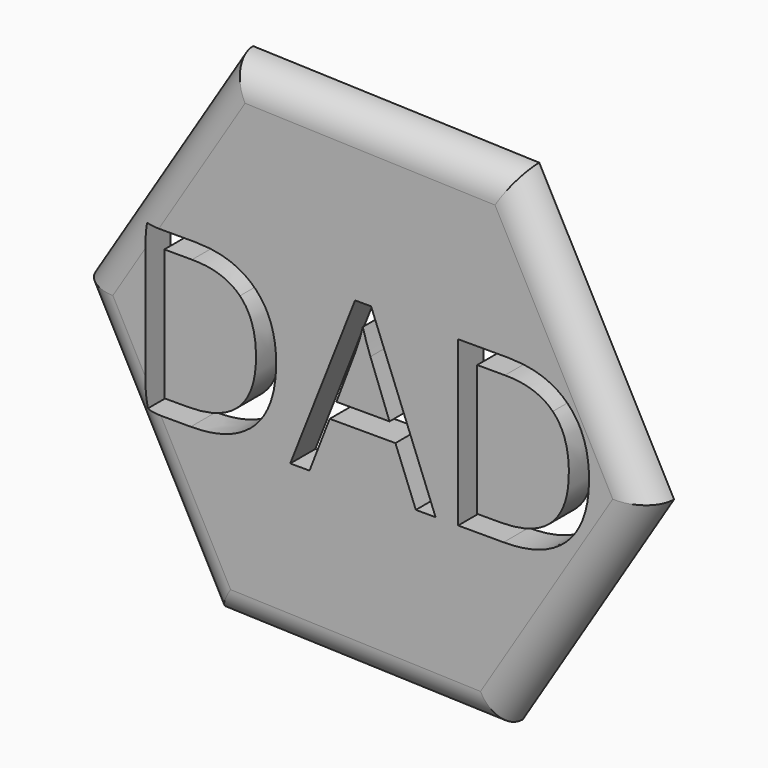
from build123d import *

# Parameters (mm, degrees)
F1_DEPTH     = 5
F2_T1_DEPTH  = 70.5879001638
F2_T3_DEPTH  = 70.5879001638
F2_T5_DEPTH  = 70.5879001638
F2_T7_DEPTH  = 70.5879001638
F2_T9_DEPTH  = 70.5879001638
F2_T11_DEPTH = 70.5879001638


# Not quite as in the source:
# - a fillet or chamfer that OpenCascade refuses, or shapes differently, is made with other operations: its cross-section is extruded or revolved along the edge and cut away or added


with BuildPart() as f1:
    # F0 (on Front) → F1 (new body)
    with BuildSketch(Plane.XZ):
        with BuildLine():
            Line((-4.1963754653, -1.9962660098), (4.2509359723, -1.9962660098))
            Line((4.2509359723, -1.9962660098), (1.2103610841, 6.0966927153))
            add(Edge.make_bspline(
                [(1.2103610841, 6.0966927153), (0.621678352, 7.6341262584), (-0.0012965781, 9.8631191276)],
                knots=[0, 0, 0, 1, 1, 1], degree=2))
            add(Edge.make_bspline(
                [(-0.0012965781, 9.8631191276), (-0.395656855, 8.1485092282), (-1.1272237454, 6.0966927153)],
                knots=[0, 0, 0, 1, 1, 1], degree=2))
            Line((-1.1272237454, 6.0966927153), (-4.1963754653, -1.9962660098))
        make_face()
    extrude(amount=F1_DEPTH)


with BuildPart() as f1b:
    # F0 (on Front) → F1, piece 2 (new body)
    with BuildSketch(Plane.XZ):
        with BuildLine():
            add(Edge.make_bspline(
                [(30.0758187402, -7.7373514895), (32.8106215297, -5.0654177297), (32.8106215297, 0.1641424634)],
                knots=[0, 0, 0, 1, 1, 1], degree=2))
            add(Edge.make_bspline(
                [(32.8106215297, 0.1641424634), (32.8106215297, 5.2736799636), (30.2472797301, 7.8627409117)],
                knots=[0, 0, 0, 1, 1, 1], degree=2))
            add(Edge.make_bspline(
                [(30.2472797301, 7.8627409117), (27.6839379305, 10.4518018597), (22.6258387274, 10.4518018597)],
                knots=[0, 0, 0, 1, 1, 1], degree=2))
            Line((22.6258387274, 10.4518018597), (18.2135759196, 10.4518018597))
            Line((18.2135759196, 10.4518018597), (18.2135759196, -10.4092852494))
            Line((18.2135759196, -10.4092852494), (21.911417936, -10.4092852494))
            add(Edge.make_bspline(
                [(21.911417936, -10.4092852494), (27.3410159507, -10.4092852494), (30.0758187402, -7.7373514895)],
                knots=[0, 0, 0, 1, 1, 1], degree=2))
        make_face()
    extrude(amount=F1_DEPTH)


with BuildPart() as f1c:
    # F0 (on Front) → F1, piece 3 (new body)
    with BuildSketch(Plane.XZ):
        Polygon((45.5624192078, -1.5240069806), (24.1010383647, 38.6962090015), (-21.4613808431, 40.2202159821), (-45.5624192078, 1.5240069806), (-24.1010383647, -38.6962090015), (21.4613808431, -40.2202159821), align=None)
        with BuildLine():
            add(Edge.make_bspline(
                [(-17.1673993541, 9.7059465535), (-13.7924755355, 6.3310227349), (-13.7924755355, 0.2727344237)],
                knots=[0, 0, 0, 1, 1, 1], degree=2))
            add(Edge.make_bspline(
                [(-13.7924755355, 0.2727344237), (-13.7924755355, -6.1913448969), (-17.3017104629, -9.6119916462)],
                knots=[0, 0, 0, 1, 1, 1], degree=2))
            add(Edge.make_bspline(
                [(-17.3017104629, -9.6119916462), (-20.8109453903, -13.0326383955), (-27.4007627703, -13.0326383955)],
                knots=[0, 0, 0, 1, 1, 1], degree=2))
            Line((-27.4007627703, -13.0326383955), (-34.6364165456, -13.0326383955))
            Line((-34.6364165456, -13.0326383955), (-34.6364165456, 13.0808703721))
            Line((-34.6364165456, 13.0808703721), (-26.6349036819, 13.0808703721))
            add(Edge.make_bspline(
                [(-26.6349036819, 13.0808703721), (-20.5423231727, 13.0808703721), (-17.1673993541, 9.7059465535)],
                knots=[0, 0, 0, 1, 1, 1], degree=2))
        make_face(mode=Mode.SUBTRACT)
        Polygon((11.5894663417, -13.0326383955), (8.4460148595, -13.0326383955), (5.193971417, -4.7282111161), (-5.2708643356, -4.7282111161), (-8.4829002137, -13.0326383955), (-11.5577673, -13.0326383955), (-1.2358157057, 13.1894623324), (1.3189530444, 13.1894623324), align=None, mode=Mode.SUBTRACT)
        with BuildLine():
            add(Edge.make_bspline(
                [(32.6477335892, 9.7059465535), (36.0226574079, 6.3310227349), (36.0226574079, 0.2727344237)],
                knots=[0, 0, 0, 1, 1, 1], degree=2))
            add(Edge.make_bspline(
                [(36.0226574079, 0.2727344237), (36.0226574079, -6.1913448969), (32.5134224805, -9.6119916462)],
                knots=[0, 0, 0, 1, 1, 1], degree=2))
            add(Edge.make_bspline(
                [(32.5134224805, -9.6119916462), (29.0041875531, -13.0326383955), (22.4143701731, -13.0326383955)],
                knots=[0, 0, 0, 1, 1, 1], degree=2))
            Line((22.4143701731, -13.0326383955), (15.1787163977, -13.0326383955))
            Line((15.1787163977, -13.0326383955), (15.1787163977, 13.0808703721))
            Line((15.1787163977, 13.0808703721), (23.1802292615, 13.0808703721))
            add(Edge.make_bspline(
                [(23.1802292615, 13.0808703721), (29.2728097706, 13.0808703721), (32.6477335892, 9.7059465535)],
                knots=[0, 0, 0, 1, 1, 1], degree=2))
        make_face(mode=Mode.SUBTRACT)
    extrude(amount=F1_DEPTH)

    # F2: fillet of radius 5 on 6 edges, made by hand

    # F2_s2 → F2_t1 (cut)
    with BuildSketch(Plane(origin=(18.6589169913, 0, 29.9584333551), x_dir=(0, 1, 0), z_dir=(-0.5286718247, 0, -0.8488263084))):
        with BuildLine():
            ThreePointArc((0, -39.480279647), (-3.5355339059, -38.015813553), (-5, -34.480279647))
            Line((-5, -34.480279647), (-5, -39.480279647))
            Line((-5, -39.480279647), (0, -39.480279647))
        make_face()
    extrude(amount=F2_T1_DEPTH, mode=Mode.SUBTRACT)

    # F2_s4 → F2_t3 (cut)
    with BuildSketch(Plane(origin=(35.2742228388, 0, -1.179879444), x_dir=(0, 1, 0), z_dir=(-0.9994410588, 0, 0.0334300763))):
        with BuildLine():
            ThreePointArc((0, -39.480279647), (-3.5355339059, -38.015813553), (-5, -34.480279647))
            Line((-5, -34.480279647), (-5, -39.480279647))
            Line((-5, -39.480279647), (0, -39.480279647))
        make_face()
    extrude(amount=F2_T3_DEPTH, mode=Mode.SUBTRACT)

    # F2_s6 → F2_t5 (cut)
    with BuildSketch(Plane(origin=(16.6153058475, 0, -31.1383127992), x_dir=(0, 1, 0), z_dir=(-0.4707692341, 0, 0.8822563846))):
        with BuildLine():
            ThreePointArc((0, -39.480279647), (-3.5355339059, -38.015813553), (-5, -34.480279647))
            Line((-5, -34.480279647), (-5, -39.480279647))
            Line((-5, -39.480279647), (0, -39.480279647))
        make_face()
    extrude(amount=F2_T5_DEPTH, mode=Mode.SUBTRACT)

    # F2_s8 → F2_t7 (cut)
    with BuildSketch(Plane(origin=(-18.6589169913, 0, -29.9584333551), x_dir=(0, 1, 0), z_dir=(0.5286718247, 0, 0.8488263084))):
        with BuildLine():
            ThreePointArc((0, -39.480279647), (-3.5355339059, -38.015813553), (-5, -34.480279647))
            Line((-5, -34.480279647), (-5, -39.480279647))
            Line((-5, -39.480279647), (0, -39.480279647))
        make_face()
    extrude(amount=F2_T7_DEPTH, mode=Mode.SUBTRACT)

    # F2_s10 → F2_t9 (cut)
    with BuildSketch(Plane(origin=(-16.6153058475, 0, 31.1383127992), x_dir=(0, 1, 0), z_dir=(0.4707692341, 0, -0.8822563846))):
        with BuildLine():
            ThreePointArc((0, -39.480279647), (-3.5355339059, -38.015813553), (-5, -34.480279647))
            Line((-5, -34.480279647), (-5, -39.480279647))
            Line((-5, -39.480279647), (0, -39.480279647))
        make_face()
    extrude(amount=F2_T9_DEPTH, mode=Mode.SUBTRACT)

    # F2_s12 → F2_t11 (cut)
    with BuildSketch(Plane(origin=(-35.2742228388, 0, 1.179879444), x_dir=(0, 1, 0), z_dir=(0.9994410588, 0, -0.0334300763))):
        with BuildLine():
            ThreePointArc((0, -39.480279647), (-3.5355339059, -38.015813553), (-5, -34.480279647))
            Line((-5, -34.480279647), (-5, -39.480279647))
            Line((-5, -39.480279647), (0, -39.480279647))
        make_face()
    extrude(amount=F2_T11_DEPTH, mode=Mode.SUBTRACT)


with BuildPart() as f1d:
    # F0 (on Front) → F1, piece 4 (new body)
    with BuildSketch(Plane.XZ):
        with BuildLine():
            add(Edge.make_bspline(
                [(-19.7393142032, -7.7373514895), (-17.0045114137, -5.0654177297), (-17.0045114137, 0.1641424634)],
                knots=[0, 0, 0, 1, 1, 1], degree=2))
            add(Edge.make_bspline(
                [(-17.0045114137, 0.1641424634), (-17.0045114137, 5.2736799636), (-19.5678532132, 7.8627409117)],
                knots=[0, 0, 0, 1, 1, 1], degree=2))
            add(Edge.make_bspline(
                [(-19.5678532132, 7.8627409117), (-22.1311950128, 10.4518018597), (-27.189294216, 10.4518018597)],
                knots=[0, 0, 0, 1, 1, 1], degree=2))
            Line((-27.189294216, 10.4518018597), (-31.6015570237, 10.4518018597))
            Line((-31.6015570237, 10.4518018597), (-31.6015570237, -10.4092852494))
            Line((-31.6015570237, -10.4092852494), (-27.9037150074, -10.4092852494))
            add(Edge.make_bspline(
                [(-27.9037150074, -10.4092852494), (-22.4741169927, -10.4092852494), (-19.7393142032, -7.7373514895)],
                knots=[0, 0, 0, 1, 1, 1], degree=2))
        make_face()
    extrude(amount=F1_DEPTH)


solid = Compound([f1.part, f1b.part, f1c.part, f1d.part])
